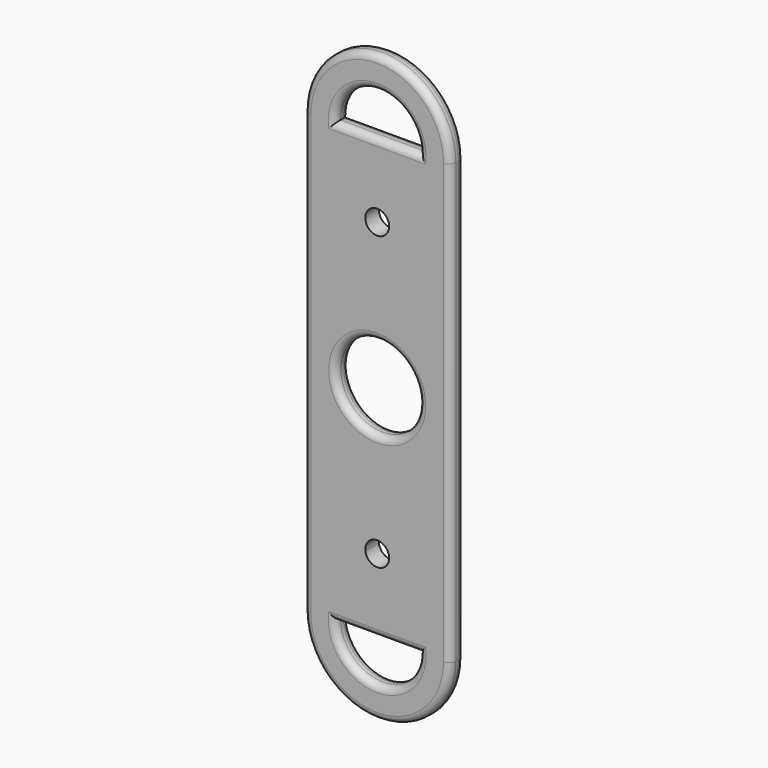
from build123d import *

# Parameters (mm, degrees)
F0_W     = 12.36
F0_H     = 4.61
F0_R     = 1
F0_R_2   = 1.75
F1_DEPTH = 2.5
F2_R     = 6.1205689933
F3_DEPTH = 25
F4_R     = 1


# Not quite as in the source:
# - a feature names something its author has since deleted; it is built from what else it names


with BuildPart() as f1:
    # F0 (on Front) → F1 (new body)
    with BuildSketch(Plane.XZ):
        with BuildLine():
            ThreePointArc((10.74, -48.33), (9.5320721777, -43.3815456959), (6.18, -39.5461967235))
            Line((6.18, -39.5461967235), (6.18, -43.72))
            Line((6.18, -43.72), (6.18, -48.33))
            ThreePointArc((6.18, -48.33), (0, -54.51), (-6.18, -48.33))
            Line((-6.18, -48.33), (-6.18, -43.72))
            Line((-6.18, -43.72), (-6.18, -39.5461967235))
            ThreePointArc((-6.18, -39.5461967235), (-9.5320721777, -43.3815456959), (-10.74, -48.33))
            ThreePointArc((-10.74, -48.33), (0, -59.07), (10.74, -48.33))
        make_face()
        with BuildLine():
            Line((6.18, 5.32), (6.18, -11.5))
            Line((6.18, -11.5), (6.18, -16.11))
            Line((6.18, -16.11), (6.18, -20.72))
            Line((6.18, -20.72), (6.18, -37.54))
            Line((6.18, -37.54), (6.18, -39.5461967235))
            ThreePointArc((6.18, -39.5461967235), (9.5320721777, -43.3815456959), (10.74, -48.33))
            Line((10.74, -48.33), (10.74, -18.9998085575))
            Line((10.74, -18.9998085575), (10.74, 16.11))
            ThreePointArc((10.74, 16.11), (0, 26.85), (-10.74, 16.11))
            Line((-10.74, 16.11), (-10.74, -18.9998085575))
            Line((-10.74, -18.9998085575), (-10.74, -48.33))
            ThreePointArc((-10.74, -48.33), (-9.5320721777, -43.3815456959), (-6.18, -39.5461967235))
            Line((-6.18, -39.5461967235), (-6.18, -37.54))
            Line((-6.18, -37.54), (-6.18, -20.72))
            Line((-6.18, -20.72), (-6.18, -16.11))
            Line((-6.18, -16.11), (-6.18, -11.5))
            Line((-6.18, -11.5), (-6.18, 5.32))
            Line((-6.18, 5.32), (-6.18, 11.5))
            Line((-6.18, 11.5), (-6.18, 16.11))
            ThreePointArc((-6.18, 16.11), (0, 22.29), (6.18, 16.11))
            Line((6.18, 16.11), (6.18, 11.5))
            Line((6.18, 11.5), (6.18, 5.32))
        make_face()
        with Locations((0, -13.805)):
            Rectangle(F0_W, F0_H)
        with Locations((0, -13.805)):
            Circle(F0_R, mode=Mode.SUBTRACT)
        with BuildLine():
            Line((-6.18, -11.5), (6.18, -11.5))
            Line((6.18, -11.5), (6.18, 5.32))
            ThreePointArc((6.18, 5.32), (0, -0.86), (-6.18, 5.32))
            Line((-6.18, 5.32), (-6.18, -11.5))
        make_face()
        with BuildLine():
            Line((6.18, -39.5461967235), (6.18, -37.54))
            ThreePointArc((6.18, -37.54), (6.1111223941, -38.4600994968), (5.9060248919, -39.3596895273))
            ThreePointArc((5.9060248919, -39.3596895273), (6.0437319312, -39.451886217), (6.18, -39.5461967235))
        make_face()
        with BuildLine():
            Line((6.18, -37.54), (6.18, -20.72))
            Line((6.18, -20.72), (-6.18, -20.72))
            Line((-6.18, -20.72), (-6.18, -37.54))
            ThreePointArc((-6.18, -37.54), (0, -31.36), (6.18, -37.54))
        make_face()
        with Locations((0, -23.415)):
            Circle(F0_R, mode=Mode.SUBTRACT)
        with BuildLine():
            Line((6.18, -43.72), (6.18, -39.5461967235))
            ThreePointArc((6.18, -39.5461967235), (6.0437319312, -39.451886217), (5.9060248919, -39.3596895273))
            ThreePointArc((5.9060248919, -39.3596895273), (4.8051050355, -41.4263048771), (3.0143614581, -42.935))
            ThreePointArc((3.0143614581, -42.935), (3.5866515341, -43.2972740217), (4.11585957, -43.72))
            Line((4.11585957, -43.72), (6.18, -43.72))
        make_face()
        with BuildLine():
            ThreePointArc((4.11585957, -43.72), (3.5866515341, -43.2972740217), (3.0143614581, -42.935))
            ThreePointArc((3.0143614581, -42.935), (1.5574498387, -43.5205309129), (0, -43.72))
            Line((0, -43.72), (4.11585957, -43.72))
        make_face()
        with BuildLine():
            Line((-6.18, -48.33), (6.18, -48.33))
            ThreePointArc((6.18, -48.33), (5.6404083249, -45.8044913525), (4.11585957, -43.72))
            Line((4.11585957, -43.72), (0, -43.72))
            Line((0, -43.72), (-4.11585957, -43.72))
            ThreePointArc((-4.11585957, -43.72), (-5.6404083249, -45.8044913525), (-6.18, -48.33))
        make_face()
        with Locations((0, -46.025)):
            Circle(F0_R, mode=Mode.SUBTRACT)
        with BuildLine():
            Line((-4.11585957, -43.72), (-6.18, -43.72))
            Line((-6.18, -43.72), (-6.18, -48.33))
            ThreePointArc((-6.18, -48.33), (-5.6404083249, -45.8044913525), (-4.11585957, -43.72))
        make_face()
        with BuildLine():
            Line((6.18, -48.33), (6.18, -43.72))
            Line((6.18, -43.72), (4.11585957, -43.72))
            ThreePointArc((4.11585957, -43.72), (5.6404083249, -45.8044913525), (6.18, -48.33))
        make_face()
        with Locations((0, -18.415)):
            Rectangle(F0_W, F0_H)
        with Locations((0, -46.025)):
            Circle(F0_R)
        with BuildLine():
            ThreePointArc((-5.9060248919, -39.3596895273), (-6.0437319312, -39.451886217), (-6.18, -39.5461967235))
            Line((-6.18, -39.5461967235), (-6.18, -43.72))
            Line((-6.18, -43.72), (-4.11585957, -43.72))
            ThreePointArc((-4.11585957, -43.72), (-3.5866515341, -43.2972740217), (-3.0143614581, -42.935))
            ThreePointArc((-3.0143614581, -42.935), (-4.8051050355, -41.4263048771), (-5.9060248919, -39.3596895273))
        make_face()
        with BuildLine():
            ThreePointArc((0, -43.72), (-1.5574498387, -43.5205309129), (-3.0143614581, -42.935))
            ThreePointArc((-3.0143614581, -42.935), (-3.5866515341, -43.2972740217), (-4.11585957, -43.72))
            Line((-4.11585957, -43.72), (0, -43.72))
        make_face()
        with BuildLine():
            ThreePointArc((5.9060248919, -39.3596895273), (6.1111223941, -38.4600994968), (6.18, -37.54))
            ThreePointArc((6.18, -37.54), (0, -31.36), (-6.18, -37.54))
            ThreePointArc((-6.18, -37.54), (-6.1111223941, -38.4600994968), (-5.9060248919, -39.3596895273))
            ThreePointArc((-5.9060248919, -39.3596895273), (-3.9084343733, -38.3264136056), (-1.7394578299, -37.7317979611))
            ThreePointArc((-1.7394578299, -37.7317979611), (-0.0960437338, -35.7926375301), (1.75, -37.54))
            ThreePointArc((1.75, -37.54), (1.7473624699, -37.6360437338), (1.7394578299, -37.7317979611))
            ThreePointArc((1.7394578299, -37.7317979611), (3.9084343733, -38.3264136056), (5.9060248919, -39.3596895273))
        make_face()
        with BuildLine():
            ThreePointArc((3.0143614581, -42.935), (4.8051050355, -41.4263048771), (5.9060248919, -39.3596895273))
            ThreePointArc((5.9060248919, -39.3596895273), (3.9084343733, -38.3264136056), (1.7394578299, -37.7317979611))
            ThreePointArc((1.7394578299, -37.7317979611), (0, -39.29), (-1.7394578299, -37.7317979611))
            ThreePointArc((-1.7394578299, -37.7317979611), (-3.9084343733, -38.3264136056), (-5.9060248919, -39.3596895273))
            ThreePointArc((-5.9060248919, -39.3596895273), (-4.8051050355, -41.4263048771), (-3.0143614581, -42.935))
            ThreePointArc((-3.0143614581, -42.935), (0, -42.15), (3.0143614581, -42.935))
        make_face()
        with BuildLine():
            ThreePointArc((0, -43.72), (1.5574498387, -43.5205309129), (3.0143614581, -42.935))
            ThreePointArc((3.0143614581, -42.935), (0, -42.15), (-3.0143614581, -42.935))
            ThreePointArc((-3.0143614581, -42.935), (-1.5574498387, -43.5205309129), (0, -43.72))
        make_face()
        with BuildLine():
            ThreePointArc((-5.9060248919, -39.3596895273), (-6.1111223941, -38.4600994968), (-6.18, -37.54))
            Line((-6.18, -37.54), (-6.18, -39.5461967235))
            ThreePointArc((-6.18, -39.5461967235), (-6.0437319312, -39.451886217), (-5.9060248919, -39.3596895273))
        make_face()
        with BuildLine():
            ThreePointArc((-6.18, 5.32), (0, -0.86), (6.18, 5.32))
            ThreePointArc((6.18, 5.32), (4.3699199077, 9.6899199077), (0, 11.5))
            ThreePointArc((0, 11.5), (-4.3699199077, 9.6899199077), (-6.18, 5.32))
        make_face()
        with Locations((0, 5.32)):
            Circle(F0_R_2, mode=Mode.SUBTRACT)
        with BuildLine():
            Line((-6.18, 11.5), (-6.18, 5.32))
            ThreePointArc((-6.18, 5.32), (-4.3699199077, 9.6899199077), (0, 11.5))
            Line((0, 11.5), (-6.18, 11.5))
        make_face()
        Polygon((0, 11.5), (6.18, 11.5), (6.18, 16.11), (-6.18, 16.11), (-6.18, 11.5), align=None)
        with Locations((0, 13.805)):
            Circle(F0_R, mode=Mode.SUBTRACT)
        with BuildLine():
            ThreePointArc((0, 11.5), (4.3699199077, 9.6899199077), (6.18, 5.32))
            Line((6.18, 5.32), (6.18, 11.5))
            Line((6.18, 11.5), (0, 11.5))
        make_face()
        with Locations((0, 13.805)):
            Circle(F0_R)
        with Locations((0, -13.805)):
            Circle(F0_R)
        with Locations((0, -23.415)):
            Circle(F0_R)
    extrude(amount=F1_DEPTH)

    # F2 (on face) → F3 (cut)
    with BuildSketch(Plane.XZ.offset(2.5)):
        with Locations((0, -16.11)):
            Circle(F2_R)
    extrude(amount=-F3_DEPTH, mode=Mode.SUBTRACT)

    # F4
    f4_edges = [f1.edges().sort_by_distance(p)[0] for p in [
        (10.74, -2.5, -16.11),
        (0, -2.5, 26.85),
        (-6.120569, -2.5, -16.11),
        (0, -2.5, 16.11),
        (0, -2.5, 22.29),
        (0, -2.5, -48.33),
        (0, -2.5, -54.51),
        (-10.74, 0, -16.11),
        (0, 0, -54.51),
        (0, 0, -48.33),
        (0, 0, 22.29),
        (0, 0, 16.11),
        (-6.120569, 0, -16.11),
    ]]
    fillet(f4_edges, radius=F4_R)


solid = f1.part
